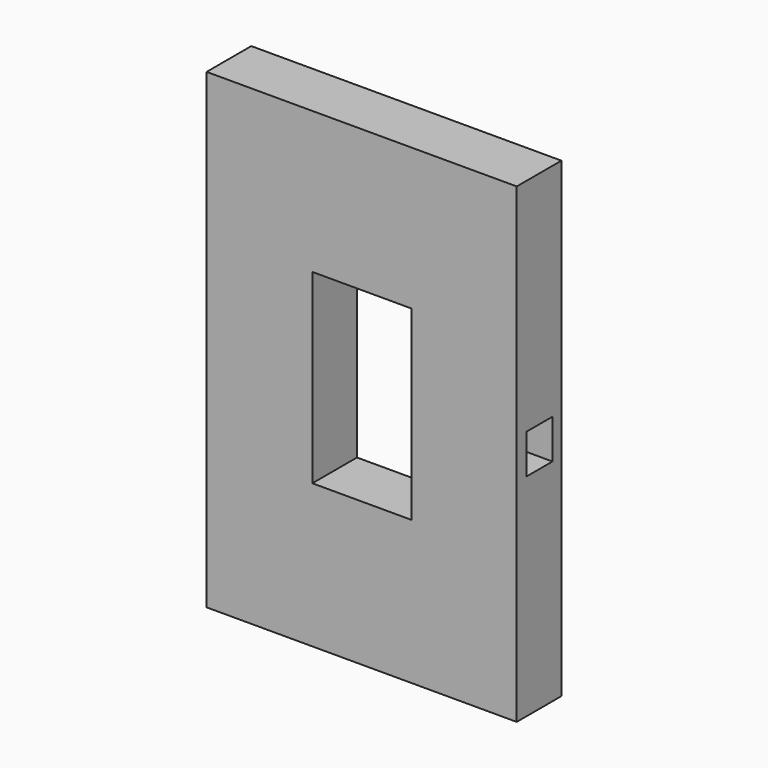
from build123d import *

# Parameters (mm, degrees)
F0_W     = 8
F0_H     = 15
F1_DEPTH = 4.5
F2_W     = 0.9
F2_H     = 3.18
F2_W_2   = 1
F3_DEPTH = 2.7


# Not quite as in the source:
# - a feature names something its author has since deleted; it is built from what else it names


with BuildPart() as f1:
    # F0 (on Front) → F1 (new body)
    with BuildSketch(Plane.XZ):
        Polygon((-92.1357174787, 21.691892745), (-117.1357174787, 21.691892745), (-117.1357174787, -16.308107255), (-92.1357174787, -16.308107255), (-92.1357174787, 0.7088574011), (-94.8357174787, 0.7088574011), (-94.8357174787, 3.8888574011), (-92.1357174787, 3.8888574011), align=None)
        with Locations((-104.6122670679, 2.7691081924)):
            Rectangle(F0_W, F0_H, mode=Mode.SUBTRACT)
    extrude(amount=F1_DEPTH)

    # F2 (on face) → F3 (join)
    with BuildSketch(Plane.YZ.offset(-94.8357174787)):
        with Locations((-0.45, 2.2988574011)):
            Rectangle(F2_W, F2_H)
        with Locations((-4, 2.2988574011)):
            Rectangle(F2_W_2, F2_H)
    extrude(amount=F3_DEPTH)


solid = f1.part
